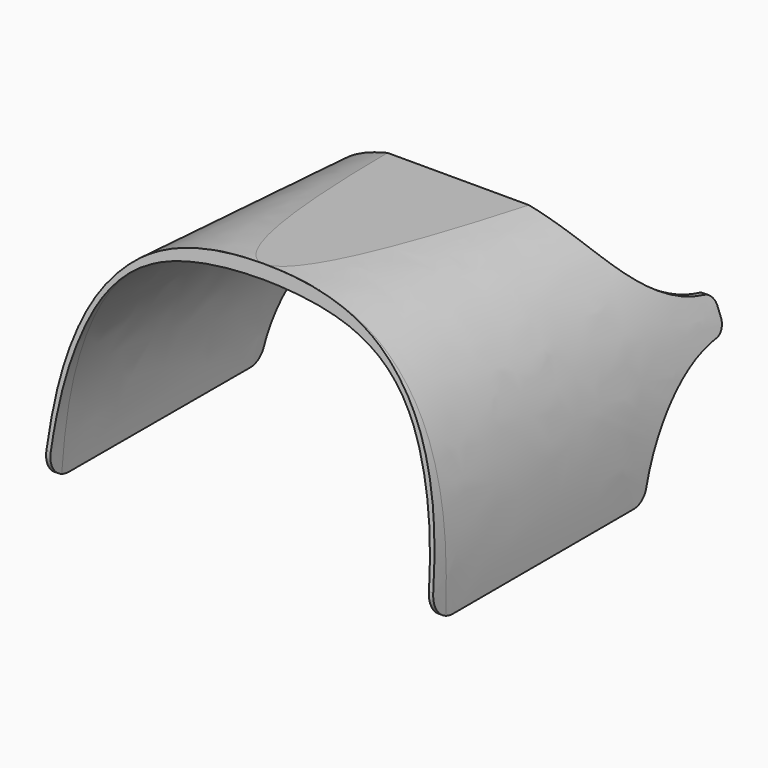
from build123d import *

# Parameters (mm, degrees)
F1_DEPTH    = 80
F4_DEPTH    = 304
F5_DEPTH    = 294
F6_T1_DEPTH = 59.2218591986
F6_T3_DEPTH = 59.2218591986
F7_R        = 7
F8_R        = 5


# Not quite as in the source:
# - a fillet or chamfer that OpenCascade refuses, or shapes differently, is made with other operations: its cross-section is extruded or revolved along the edge and cut away or added
# - a feature names something its author has since deleted; it is built from what else it names


with BuildPart() as f1:
    # F0 (on Right) → F1 (new body, symmetric)
    with BuildSketch(Plane.YZ):
        with BuildLine():
            Line((-26.1265078879, 48.2496146113), (-40.1163027436, -51.5445995849))
            Line((-40.1163027436, -51.5445995849), (69.8836972564, -51.5445995849))
            ThreePointArc((69.8836972564, -51.5445995849), (87.2507155104, -22.8147661228), (118.8734921121, -11.5445995849))
            Line((118.8734921121, -11.5445995849), (118.8734921121, 1.359343739))
            ThreePointArc((118.8734921121, 1.359343739), (91.0722509444, 13.4118882647), (73.8734921121, 38.359343739))
            Line((73.8734921121, 38.359343739), (-26.1265078879, 48.2496146113))
        make_face()
    extrude(amount=F1_DEPTH, both=True)

    # F3 (on face) → F4 (cut, symmetric)
    with BuildSketch(Plane(origin=(0, -29.0868094694, 1.8559815741), x_dir=(-1, 0, 0), z_dir=(0, 0.9979704421, -0.063678856))):
        with BuildLine():
            add(Edge.make_bspline(
                [(0, 46.4879830907), (-31.5785962088, 46.4879830907), (-58.6130435871, 30.2772286719), (-76.1504732807, -3.9774534187), (-80, -32.6448029283), (-80, -59.9699916285)],
                knots=[0, 0, 0, 0, 0.3708692756, 0.6380824372, 1, 1, 1, 1], degree=3))
            add(Edge.make_bspline(
                [(0, 46.4879830907), (31.5785962088, 46.4879830907), (58.6130435871, 30.2772286719), (76.1504732807, -3.9774534187), (80, -32.6448029283), (80, -59.9699916285)],
                knots=[0, 0, 0, 0, 0.3708692756, 0.6380824372, 1, 1, 1, 1], degree=3))
            Line((80, -59.9699916285), (133.3417594433, -11.8499875401))
            Line((133.3417594433, -11.8499875401), (48.4413430095, 102.7011049579))
            Line((48.4413430095, 102.7011049579), (-65.9957453609, 102.7011049579))
            Line((-65.9957453609, 102.7011049579), (-136.9278281927, -18.2866046537))
            Line((-136.9278281927, -18.2866046537), (-80, -59.9699916285))
        make_face()
    extrude(amount=F4_DEPTH, both=True, mode=Mode.SUBTRACT)

    # F3 (on face) → F5 (cut, symmetric)
    with BuildSketch(Plane(origin=(0, -29.0868094694, 1.8559815741), x_dir=(-1, 0, 0), z_dir=(0, 0.9979704421, -0.063678856))):
        with BuildLine():
            add(Edge.make_bspline(
                [(0, 41.1681465075), (30.2756745707, 40.9343968924), (57.3175236506, 29.603100291), (74.2541446528, -5.6979199795), (78.2161146403, -33.4861980588), (78.2977019192, -60.0071400039)],
                knots=[0.0067145844, 0.0067145844, 0.0067145844, 0.0067145844, 0.3687093588, 0.6367265715, 0.9933274262, 0.9933274262, 0.9933274262, 0.9933274262], degree=3))
            add(Edge.make_bspline(
                [(0, 41.1681465075), (-30.2756745707, 40.9343968924), (-57.3175236505, 29.603100291), (-74.2541446528, -5.6979199795), (-78.2161146403, -33.4861980588), (-78.2977019192, -60.0071400039)],
                knots=[0.0067145844, 0.0067145844, 0.0067145844, 0.0067145844, 0.3687093588, 0.6367265715, 0.9933274262, 0.9933274262, 0.9933274262, 0.9933274262], degree=3))
            Line((-78.2977019192, -60.0071400039), (78.2977019192, -60.0071400039))
        make_face()
    extrude(amount=F5_DEPTH, both=True, mode=Mode.SUBTRACT)

    # F6: fillet of radius 10 on 2 edges, made by hand

    # F6_s2 → F6_t1 (cut)
    with BuildSketch(Plane.YZ.offset(49.4897365309)):
        with BuildLine():
            ThreePointArc((-38.5198191101, -40.156310384), (-36.1626109237, -48.1065012906), (-28.6166553179, -51.5445995849))
            Line((-28.6166553179, -51.5445995849), (-40.1163027436, -51.5445995849))
            Line((-40.1163027436, -51.5445995849), (-38.5198191101, -40.156310384))
        make_face()
    extrude(amount=F6_T1_DEPTH, mode=Mode.SUBTRACT)

    # F6_s4 → F6_t3 (cut)
    with BuildSketch(Plane.YZ.offset(-108.7115957295)):
        with BuildLine():
            ThreePointArc((-38.5198191101, -40.156310384), (-36.1626109237, -48.1065012906), (-28.6166553179, -51.5445995849))
            Line((-28.6166553179, -51.5445995849), (-40.1163027436, -51.5445995849))
            Line((-40.1163027436, -51.5445995849), (-38.5198191101, -40.156310384))
        make_face()
    extrude(amount=F6_T3_DEPTH, mode=Mode.SUBTRACT)

    # F7
    f7_edges = [f1.edges().sort_by_distance(p)[0] for p in [
        (-78.93127, 69.883697, -51.5446),
        (78.93127, 69.883697, -51.5446),
    ]]
    fillet(f7_edges, radius=F7_R)

    # F8
    f8_edges = [f1.edges().sort_by_distance(p)[0] for p in [
        (67.749324, 118.873492, 1.359344),
        (-67.749324, 118.873492, 1.359344),
        (72.711952, 118.873492, -11.5446),
        (-72.711952, 118.873492, -11.5446),
    ]]
    fillet(f8_edges, radius=F8_R)


solid = f1.part
